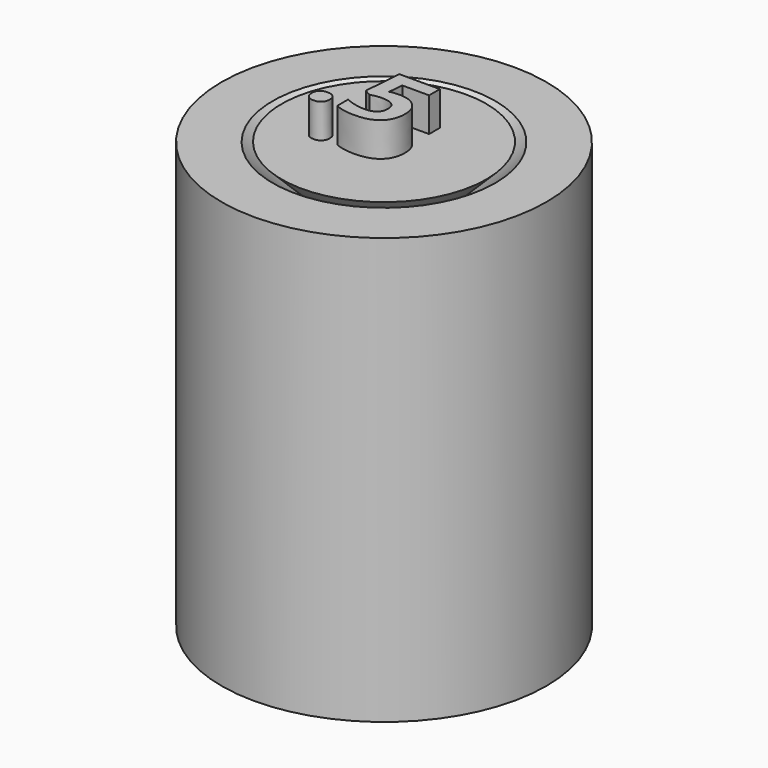
from build123d import *

# Parameters (mm, degrees)
F2_TEXT_SIZE = 6.1593815594
F3_DEPTH     = 2


# Not quite as in the source:
# - Text() gives the source's letters only with a copy of the font that has no kerning and outlines rounded to 1/6400 em; it was checked with that copy


with BuildPart() as f1:
    # F0 (on Front) → F1 (revolve)
    with BuildSketch(Plane.XZ):
        Polygon((6, 25), (0, 25), (0, 22), (0, 3), (0, 0), (6, 0), (3, 3), (3, 22), align=None)
    revolve(axis=Axis((0, 0, 12.5), (0, 0, 1)))

    # F2 (on face) → F3 (join)
    with BuildSketch(Plane.XY.offset(25)):
        with Locations((-3.5493343603, -1.7350238049)):
            Text('.5', F2_TEXT_SIZE, font='Open Sans', font_style=FontStyle.BOLD, text_align=(TextAlign.LEFT, TextAlign.BOTTOM))
    extrude(amount=F3_DEPTH)


with BuildPart() as f1b:
    # F0 (on Front) → F1, piece 2 (revolve)
    with BuildSketch(Plane.XZ):
        Polygon((6.5240137267, 24.979188137), (3.4999883892, 22.0034074398), (3.5240156792, 3.0034226322), (6.5240156792, 0.0034226322), (9.5240137267, 0), (9.5240137267, 24.979188137), align=None)
    revolve(axis=Axis((0, 0, 12.5), (0, 0, 1)))


solid = Compound([f1.part, f1b.part])
